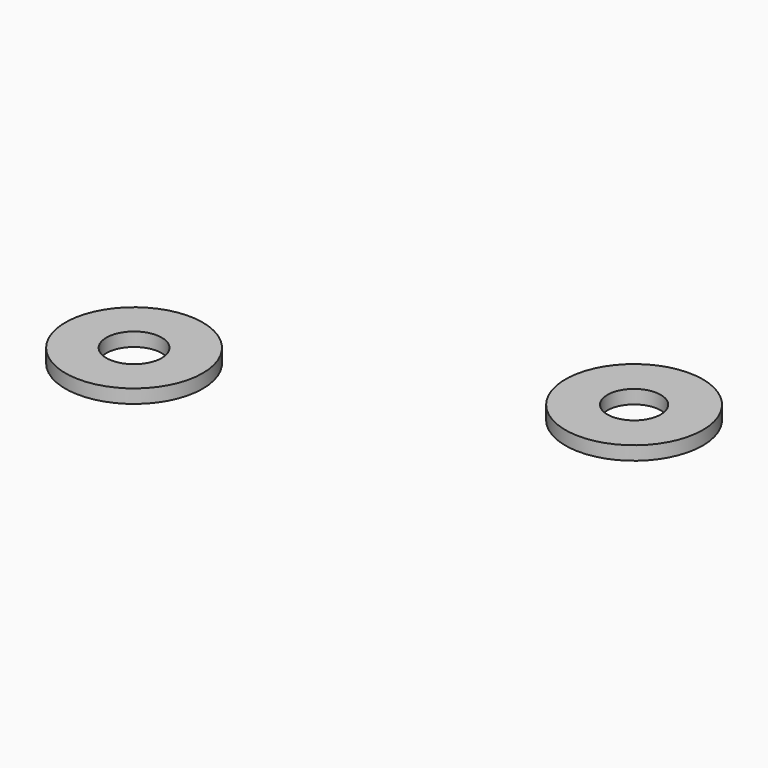
from build123d import *

# Parameters (mm, degrees)
F0_R     = 10.05
F0_R_2   = 4.05
F1_DEPTH = 2
F0_R_3   = 3.9


# Not quite as in the source:
# - the program builds the solid bodies; features that only make, move or delete a surface that nothing else refers to are left out


with BuildPart() as f1:
    # F0 (on Top) → F1 (new body)
    with BuildSketch(Plane.XY):
        with Locations((-31.974799931, 19.1264785826)):
            Circle(F0_R)
        with Locations((-31.974799931, 19.1264785826)):
            Circle(F0_R_2, mode=Mode.SUBTRACT)
    extrude(amount=F1_DEPTH)


with BuildPart() as f1b:
    # F0 (on Top) → F1, piece 2 (new body)
    with BuildSketch(Plane.XY):
        with Locations((21.411953494, 43.8298359513)):
            Circle(F0_R)
        with Locations((21.411953494, 43.8298359513)):
            Circle(F0_R_3, mode=Mode.SUBTRACT)
    extrude(amount=F1_DEPTH)


solid = Compound([f1.part, f1b.part])
